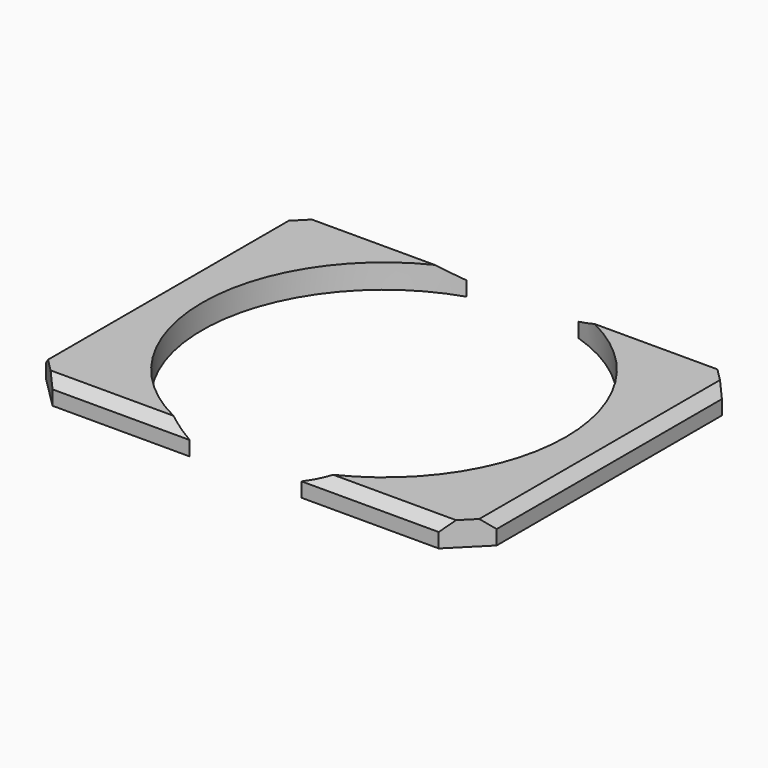
from build123d import *

# Parameters (mm, degrees)
F1_DEPTH      = 3.81
F2_SIZE       = 1.524
F2_2_SIZE     = 1.524
F3_T1_DEPTH   = 28.4142991577
F3_2_T1_DEPTH = 28.4142991577


# Not quite as in the source:
# - a fillet or chamfer that OpenCascade refuses, or shapes differently, is made with other operations: its cross-section is extruded or revolved along the edge and cut away or added


with BuildPart() as f1:
    # F0 (on Top) → F1 (new body)
    with BuildSketch(Plane.XY):
        with BuildLine():
            Line((-8.8454383159, 27.305), (-35.56, 27.305))
            Line((-35.56, 27.305), (-35.56, -27.305))
            Line((-35.56, -27.305), (-8.8454383159, -27.305))
            ThreePointArc((-8.8454383159, -27.305), (-28.702, 0), (-8.8454383159, 27.305))
        make_face()
    extrude(amount=F1_DEPTH)

    # F2
    f2_edges = [f1.edges().sort_by_distance(p)[0] for p in [
        (-35.56, 0, 3.81),
        (-22.202719, 27.305, 3.81),
        (-22.202719, -27.305, 3.81),
    ]]
    chamfer(f2_edges, length=F2_SIZE)

    # F3#2: chamfer of 5.08 on 2 edges, made by hand

    # F3_2_s2 → F3_2_t1 (cut)
    with BuildSketch(Plane.XY.offset(-13.0641495789)):
        Polygon((-35.56, -22.225), (-30.48, -27.305), (-35.56, -27.305), align=None)
        Polygon((-30.48, 27.305), (-35.56, 22.225), (-35.56, 27.305), align=None)
    extrude(amount=F3_2_T1_DEPTH, mode=Mode.SUBTRACT)


with BuildPart() as f1b:
    # F0 (on Top) → F1, piece 2 (new body)
    with BuildSketch(Plane.XY):
        with BuildLine():
            Line((35.56, 27.305), (8.8454383159, 27.305))
            ThreePointArc((8.8454383159, 27.305), (23.2129982396, 16.8808032015), (28.702, 0))
            ThreePointArc((28.702, 0), (23.2129982396, -16.8808032015), (8.8454383159, -27.305))
            Line((8.8454383159, -27.305), (35.56, -27.305))
            Line((35.56, -27.305), (35.56, 27.305))
        make_face()
    extrude(amount=F1_DEPTH)

    # F2#2
    f2_2_edges = [f1b.edges().sort_by_distance(p)[0] for p in [
        (22.202719, -27.305, 3.81),
        (35.56, 0, 3.81),
        (22.202719, 27.305, 3.81),
    ]]
    chamfer(f2_2_edges, length=F2_2_SIZE)

    # F3: chamfer of 5.08 on 2 edges, made by hand

    # F3_s2 → F3_t1 (cut)
    with BuildSketch(Plane.XY.offset(-13.0641495789)):
        Polygon((30.48, -27.305), (35.56, -22.225), (35.56, -27.305), align=None)
        Polygon((35.56, 22.225), (30.48, 27.305), (35.56, 27.305), align=None)
    extrude(amount=F3_T1_DEPTH, mode=Mode.SUBTRACT)


solid = Compound([f1.part, f1b.part])
